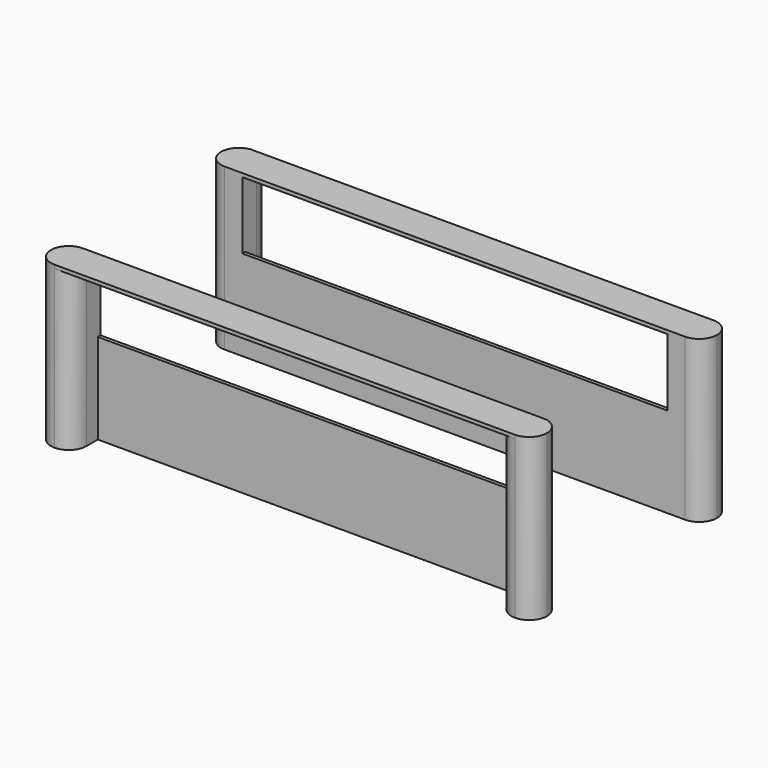
from build123d import *

# Parameters (mm, degrees)
F0_W      = 20
F0_H      = 18
F1_DEPTH  = 1
F3_DEPTH  = 50
F2_W      = 20
F2_H      = 18
F4_DEPTH  = 90
F5_W      = 20
F5_H      = 2
F6_DEPTH  = 40
F7_DEPTH  = 25
F9_R      = 9.99999
F10_W     = 9.99999
F10_H     = 2
F10_W_2   = 10.00001
F11_DEPTH = 240
F13_DEPTH = 2
F10_W_3   = 20
F14_DEPTH = 240
F12_W     = 11.77511096
F12_H     = 12.0397691429
F15_DEPTH = 2


# Not quite as in the source:
# - a fillet or chamfer is up to 0.001 mm smaller than in the source, because OpenCascade refuses the exact size
# - ends of sketch curves that miss each other by under 0.0002 mm in the source are joined
# - a feature of the source that left no trace in its solid (it failed there, or was rolled back) is left out


with BuildPart() as f1:
    # F0 (on Top) → F1 (new body)
    with BuildSketch(Plane.XY):
        with Locations((130, 59)):
            Rectangle(F0_W, F0_H)
        with Locations((-130, 59)):
            Rectangle(F0_W, F0_H)
        Polygon((-140, -70), (140, -70), (140, -68), (120, -68), (-120, -68), (-140, -68), align=None)
        with Locations((-130, -59)):
            Rectangle(F0_W, F0_H)
        Polygon((120, -50), (140, -50), (140, 50), (120, 50), (120, 68), (-120, 68), (-120, 50), (-140, 50), (-140, -50), (-120, -50), (-120, -68), (120, -68), align=None)
        Polygon((120, 68), (140, 68), (140, 70), (-140, 70), (-140, 68), (-120, 68), align=None)
        with Locations((130, -59)):
            Rectangle(F0_W, F0_H)
    extrude(amount=F1_DEPTH)

    # F2 (on face) → F3 (join)
    with BuildSketch(Plane.XY.offset(1)):
        Polygon((-140, 52), (-140, 50), (140, 50), (140, 52), (120, 52), (-120, 52), align=None)
        Polygon((-140, -50), (-140, -52), (-120, -52), (120, -52), (140, -52), (140, -50), align=None)
    extrude(amount=F3_DEPTH)

    # F2 (on face) → F4 (join)
    with BuildSketch(Plane.XY.offset(1)):
        with Locations((-130, -61)):
            Rectangle(F2_W, F2_H)
        with Locations((130, -61)):
            Rectangle(F2_W, F2_H)
        with Locations((130, 61)):
            Rectangle(F2_W, F2_H)
        with Locations((-130, 61)):
            Rectangle(F2_W, F2_H)
    extrude(amount=F4_DEPTH)

    # F5 (on face) → F6 (join)
    with BuildSketch(Plane.XY.offset(51)):
        with Locations((-130, -51)):
            Rectangle(F5_W, F5_H)
        Polygon((-140, 50), (-120, 50), (-120, 52), (-120, 52.0472601056), (-140, 52.0472601056), align=None)
        with Locations((130, -51)):
            Rectangle(F5_W, F5_H)
        with Locations((130, 51)):
            Rectangle(F5_W, F5_H)
    extrude(amount=F6_DEPTH)

    # F7 (cut): faces of the model
    f7_faces = [f1.faces().sort_by_distance(p)[0] for p in [
        (0, -61, 1),
        (0, 0, 1),
        (0, 61, 1),
    ]]
    extrude(f7_faces, amount=-F7_DEPTH, mode=Mode.SUBTRACT)

    # F9 (radius 10 in the source; OpenCascade refuses exactly that, so slightly less here)
    f9_edges = [f1.edges().sort_by_distance(p)[0] for p in [
        (140, 50, 45.5),
        (140, 70, 45.5),
        (140, -70, 45.5),
        (140, -50, 45.5),
        (120, -70, 45.5),
        (120, 70, 45.5),
        (-120, 70, 45.5),
        (-140, 50, 45.5),
        (-140, 70, 45.5),
        (-120, -70, 45.5),
        (-140, -70, 45.5),
        (-140, -50, 45.5),
    ]]
    fillet(f9_edges, radius=F9_R)

    # F10 (on face) → F11 (join)
    with BuildSketch(Plane(origin=(120, 0, 0), x_dir=(0, -1, 0), z_dir=(-1, 0, 0))):
        with Locations((65.000005, 90)):
            Rectangle(F10_W, F10_H)
        with Locations((55.000005, 90)):
            Rectangle(F10_W_2, F10_H)
    extrude(amount=F11_DEPTH)

    # F12 (on face) → F13 (join)
    with BuildSketch(Plane.XY.offset(91)):
        with BuildLine():
            Line((-130, -70), (-120, -70))
            Line((-120, -70), (-120, -60.00001))
            ThreePointArc((-120, -60.00001), (-122.9289292592, -67.0710707408), (-130, -70))
        make_face()
        with BuildLine():
            Line((120, -60.00001), (120, -70))
            Line((120, -70), (130, -70))
            ThreePointArc((130, -70), (122.9289292592, -67.0710707408), (120, -60.00001))
        make_face()
    extrude(amount=-F13_DEPTH)

    # F10 (on face) → F14 (join)
    with BuildSketch(Plane(origin=(120, 0, 0), x_dir=(0, -1, 0), z_dir=(-1, 0, 0))):
        with Locations((-60, 90)):
            Rectangle(F10_W_3, F10_H)
    extrude(amount=F14_DEPTH)

    # F12 (on face) → F15 (join)
    with BuildSketch(Plane.XY.offset(91)):
        with Locations((125.88755548, 63.9801154286)):
            Rectangle(F12_W, F12_H)
        with Locations((-125.88755548, 63.9801154286)):
            Rectangle(F12_W, F12_H)
    extrude(amount=-F15_DEPTH)


solid = f1.part
